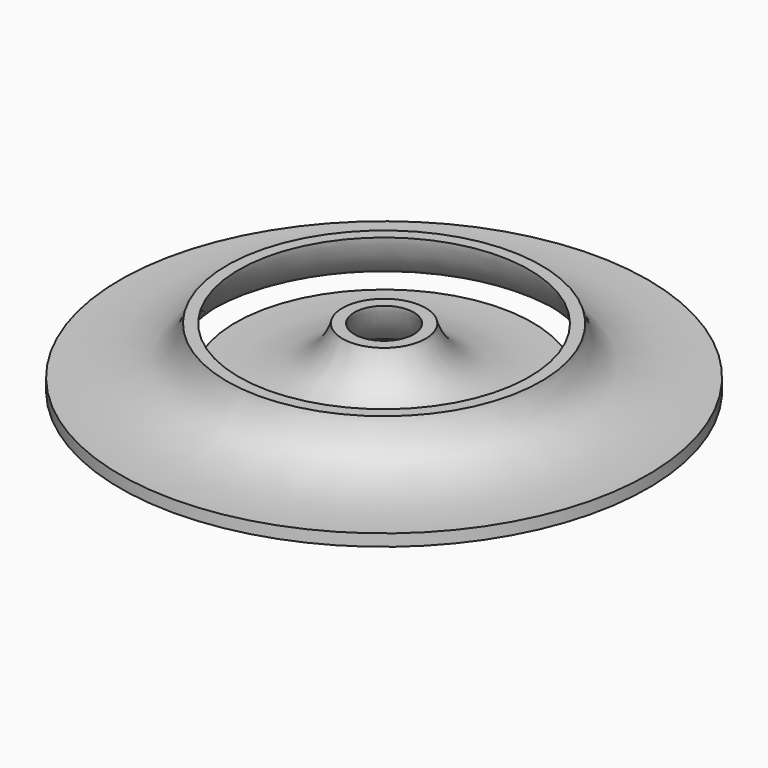
from build123d import *


# Not quite as in the source:
# - ends of sketch curves that miss each other by under 0.0002 mm in the source are joined
# - the dataset's text gives a spline's control points without its knots; the knots are read off the source's solid


with BuildPart() as f1:
    # F0 (on Right) → F1 (revolve)
    with BuildSketch(Plane.YZ):
        with BuildLine():
            Line((-25, 2), (-25, 0))
            add(Edge.make_bspline(
                [(-25, 0), (-23, 0), (-8.2428042968, -0.7589394656), (-5, 9), (-5, 10)],
                knots=[0, 0, 0, 0, 0.5650030571, 1, 1, 1, 1], degree=3))
            Line((-5, 10), (-7.0049383579, 10))
            add(Edge.make_bspline(
                [(-25, 2), (-24.8744459418, 2), (-24.6020502652, 1.997175871), (-23.944655641, 1.9866596386), (-22.9136976758, 1.9733202808), (-21.3996719503, 1.985743252), (-19.1160811737, 2.077743282), (-16.5976005336, 2.3399298707), (-14.1945196869, 2.8670138177), (-12.8187529126, 3.3179992457), (-11.8400283506, 3.7514181037), (-11.2876311756, 4.0507249853), (-10.8861388194, 4.3053949031), (-10.4981730414, 4.5778538923), (-10.0413189077, 4.9474282096), (-9.5365181247, 5.4304731797), (-8.9222342339, 6.1152949724), (-8.3975554045, 6.8420822439), (-7.9652985038, 7.5662331827), (-7.6876671922, 8.0956131465), (-7.4567771073, 8.5983270086), (-7.2726178766, 9.0603628688), (-7.1350687961, 9.4658352411), (-7.0591636163, 9.7405002539), (-7.0261213485, 9.8866268551), (-7.0128338895, 9.9538462647), (-7.0075458312, 9.9839495944), (-7.0052842517, 9.9978468696), (-7.0049383579, 10)],
                knots=[0, 0, 0, 0, 0.0310334646, 0.0620669291, 0.1241338583, 0.1862007874, 0.2482677166, 0.3724015748, 0.434468504, 0.4965354331, 0.5275688977, 0.5586023623, 0.5741190946, 0.5896358268, 0.6206692914, 0.651702756, 0.6827362205, 0.7448031497, 0.7758366143, 0.8068700788, 0.8379035434, 0.868937008, 0.8999704725, 0.9310039371, 0.9465206694, 0.9542790355, 0.9620374017, 0.9635107276, 0.9635107276, 0.9635107276, 0.9635107276], degree=3))
        make_face()
    revolve(axis=Axis((0, 0, 5), (0, 0, 1)))


with BuildPart() as f1b:
    # F0 (on Right) → F1, piece 2 (revolve)
    with BuildSketch(Plane.YZ):
        with BuildLine():
            Line((-44.4571920699, 2), (-44.4571920699, 0))
            add(Edge.make_bspline(
                [(-44.4571920699, 0), (-42.4571920699, 0), (-27.2973141645, -0.8451838413), (-24.4571920699, 9), (-24.4571920699, 10)],
                knots=[0, 0, 0, 0, 0.5690663499, 1, 1, 1, 1], degree=3))
            Line((-24.4571920699, 10), (-26.4591868733, 10))
            add(Edge.make_bspline(
                [(-44.4571920699, 2), (-44.3301263073, 2), (-44.0550017899, 1.9968187714), (-43.3885761174, 1.984637898), (-42.3388801305, 1.9677078809), (-40.7928507171, 1.9742609155), (-39.0423480087, 2.0370462661), (-37.1735164079, 2.1845748373), (-35.2766244821, 2.4434034033), (-33.4457129988, 2.8359140628), (-32.056717366, 3.2865627122), (-31.0771304396, 3.7196898786), (-30.5282614983, 4.0186874168), (-30.1335263651, 4.2717762624), (-29.7544595412, 4.5423113151), (-29.3104788796, 4.9100474895), (-28.8234660731, 5.3917736768), (-28.2348659256, 6.076381331), (-27.7378183493, 6.8052783607), (-27.3332027443, 7.5329427062), (-27.0757776785, 8.0652700313), (-26.863973887, 8.5708812724), (-26.6971113951, 9.0354330637), (-26.5743133468, 9.4428196945), (-26.5078615414, 9.7185644574), (-26.4795083628, 9.8653164013), (-26.4682793946, 9.9328847921), (-26.4625155073, 9.9725570807), (-26.4600673639, 9.9923272701), (-26.4591868733, 10)],
                knots=[0, 0, 0, 0, 0.0311589612, 0.0623179224, 0.1246358447, 0.1869537671, 0.2492716894, 0.3115896118, 0.3739075342, 0.4362254565, 0.4985433789, 0.5297023401, 0.5608613012, 0.5764407818, 0.5920202624, 0.6231792236, 0.6543381848, 0.685497146, 0.7478150683, 0.7789740295, 0.8101329907, 0.8412919518, 0.872450913, 0.9036098742, 0.9347688354, 0.950348316, 0.9581380563, 0.9659277966, 0.9726893525, 0.9726893525, 0.9726893525, 0.9726893525], degree=3))
        make_face()
    revolve(axis=Axis((0, 0, 5), (0, 0, 1)))


solid = Compound([f1.part, f1b.part])
